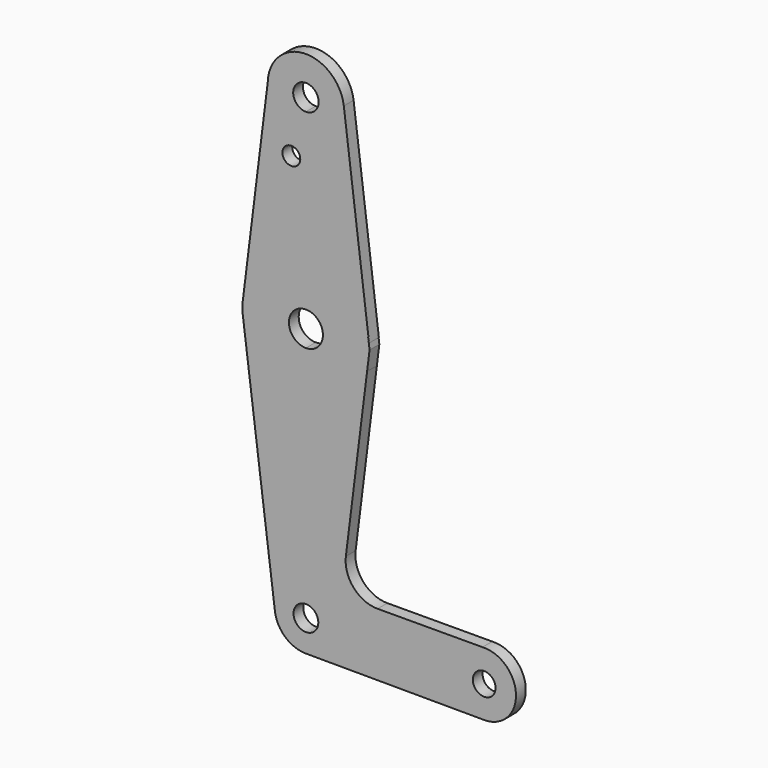
from build123d import *

# Parameters (mm, degrees)
F0_R     = 2.2225
F1_DEPTH = 3.048


# Not quite as in the source:
# - ends of sketch curves that miss each other by under 0.0002 mm in the source are joined


with BuildPart() as f1:
    # F0 (on Front) → F1 (new body)
    with BuildSketch(Plane.XZ):
        with BuildLine():
            Line((0, 104.775), (0, 79.375))
            ThreePointArc((0, 79.375), (9.9062001273, 75.9049515935), (15.4816923534, 67.0118124772))
            ThreePointArc((15.4816923534, 67.0118124772), (15.634754331, 66.2513782015), (15.7504882737, 65.484375))
            Line((15.7504882737, 65.484375), (9.4502929642, 115.490625))
            ThreePointArc((9.4502929642, 115.490625), (9.5063048942, 114.896483242), (9.525, 114.3))
            ThreePointArc((9.525, 114.3), (6.7351920908, 107.5648079092), (0, 104.775))
        make_face()
        with BuildLine():
            ThreePointArc((-15.3768101201, 67.4457997325), (-9.7307773134, 76.0430298523), (0, 79.375))
            Line((0, 79.375), (0, 104.775))
            ThreePointArc((0, 104.775), (-6.8164586923, 107.6470671207), (-9.5221925783, 114.5312433813))
            Line((-9.5221925783, 114.5312433813), (-15.3768101201, 67.4457997325))
        make_face()
        with Locations((-3.6322334781, 100.2735868096)):
            Circle(F0_R, mode=Mode.SUBTRACT)
        with BuildLine():
            ThreePointArc((-9.5221925783, 114.5312433813), (-6.8164586923, 107.6470671207), (0, 104.775))
            ThreePointArc((0, 104.775), (6.7351920908, 107.5648079092), (9.525, 114.3))
            ThreePointArc((9.525, 114.3), (9.5063048942, 114.896483242), (9.4502929642, 115.490625))
            ThreePointArc((9.4502929642, 115.490625), (-0.481036029, 123.8128454912), (-9.5221925783, 114.5312433813))
        make_face()
        with BuildLine():
            ThreePointArc((3.1731383542, 114.3), (2.2437476479, 112.0562523521), (0, 111.1268616458))
            ThreePointArc((0, 111.1268616458), (-2.2437476479, 116.5437476479), (3.1731383542, 114.3))
        make_face(mode=Mode.SUBTRACT)
        with BuildLine():
            Line((0, 59.2630050683), (0, 47.625))
            ThreePointArc((0, 47.625), (9.5420870367, 50.8128332563), (15.2519117252, 59.0960456714))
            Line((15.2519117252, 59.0960456714), (15.8668198703, 64.0095607934))
            Line((15.8668198703, 64.0095607934), (15.4816923534, 67.0118124772))
            ThreePointArc((15.4816923534, 67.0118124772), (9.9062001273, 75.9049515935), (0, 79.375))
            Line((0, 79.375), (0, 67.7369949317))
            ThreePointArc((0, 67.7369949317), (2.996007848, 66.496007848), (4.2369949317, 63.5))
            ThreePointArc((4.2369949317, 63.5), (2.996007848, 60.503992152), (0, 59.2630050683))
        make_face()
        with BuildLine():
            ThreePointArc((-15.7459735632, 61.4801134818), (-10.4868948341, 51.5819187057), (0, 47.625))
            Line((0, 47.625), (0, 59.2630050683))
            ThreePointArc((0, 59.2630050683), (-4.2369949317, 63.5), (0, 67.7369949317))
            Line((0, 67.7369949317), (0, 79.375))
            ThreePointArc((0, 79.375), (-9.7307773134, 76.0430298523), (-15.3768101201, 67.4457997325))
            Line((-15.3768101201, 67.4457997325), (-15.8748867846, 63.4400452066))
            ThreePointArc((-15.8748867846, 63.4400452066), (-15.8407712999, 62.4580836766), (-15.7459735632, 61.4801134818))
        make_face()
        with BuildLine():
            ThreePointArc((-7.7320952095, -0.9918697506), (-5.8524002287, 5.1496129461), (0, 7.7954539272))
            Line((0, 7.7954539272), (0, 47.625))
            ThreePointArc((0, 47.625), (-10.4868948341, 51.5819187057), (-15.7459735632, 61.4801134818))
            Line((-15.7459735632, 61.4801134818), (-7.7320952095, -0.9918697506))
        make_face()
        with BuildLine():
            Line((0, 47.625), (0, 7.7954539272))
            ThreePointArc((0, 7.7954539272), (5.5122183343, 5.5122183343), (7.7954539272, 0))
            Line((7.7954539272, 0), (36.5125, 0))
            ThreePointArc((36.5125, 0), (38.6941635505, 5.4657344444), (44.0398708389, 7.9268972695))
            Line((44.0398708389, 7.9268972695), (17.869380753, 7.8488082918))
            ThreePointArc((17.869380753, 7.8488082918), (11.8930439791, 10.5290526777), (9.9569931381, 16.7862100471))
            Line((9.9569931381, 16.7862100471), (15.2519117252, 59.0960456714))
            ThreePointArc((15.2519117252, 59.0960456714), (9.5420870367, 50.8128332563), (0, 47.625))
        make_face()
        with BuildLine():
            Line((36.5125, 0), (7.7954539272, 0))
            ThreePointArc((7.7954539272, 0), (5.5122183343, -5.5122183343), (0, -7.7954539272))
            Line((0, -7.7954539272), (43.9269950713, -7.9202507596))
            ThreePointArc((43.9269950713, -7.9202507596), (38.6553793104, -5.4245992768), (36.5125, 0))
        make_face()
        with BuildLine():
            ThreePointArc((3.0872431229, 0), (-2.1830105474, -2.1830105474), (0, 3.0872431229))
            Line((0, 3.0872431229), (0, 7.7954539272))
            ThreePointArc((0, 7.7954539272), (-5.8524002287, 5.1496129461), (-7.7320952095, -0.9918697506))
            ThreePointArc((-7.7320952095, -0.9918697506), (-5.1496129461, -5.8524002287), (0, -7.7954539272))
            ThreePointArc((0, -7.7954539272), (5.5122183343, -5.5122183343), (7.7954539272, 0))
            Line((7.7954539272, 0), (3.0872431229, 0))
        make_face()
        with BuildLine():
            Line((0, 7.7954539272), (0, 3.0872431229))
            ThreePointArc((0, 3.0872431229), (2.1830105474, 2.1830105474), (3.0872431229, 0))
            Line((3.0872431229, 0), (7.7954539272, 0))
            ThreePointArc((7.7954539272, 0), (5.5122183343, 5.5122183343), (0, 7.7954539272))
        make_face()
        with BuildLine():
            ThreePointArc((44.0398708389, 7.9268972695), (38.6941635505, 5.4657344444), (36.5125, 0))
            ThreePointArc((36.5125, 0), (38.6553793104, -5.4245992768), (43.9269950713, -7.9202507596))
            Line((43.9269950713, -7.9202507596), (44.9280052412, -7.9230939184))
            ThreePointArc((44.9280052412, -7.9230939184), (50.2291899455, -5.4410357308), (52.3875, 0))
            ThreePointArc((52.3875, 0), (49.9157344444, 5.7558364495), (44.0398708389, 7.9268972695))
        make_face()
        with BuildLine():
            ThreePointArc((47.2789731749, 0), (44.45, -2.8289731749), (41.6210268251, 0))
            ThreePointArc((41.6210268251, 0), (44.45, 2.8289731749), (47.2789731749, 0))
        make_face(mode=Mode.SUBTRACT)
    extrude(amount=F1_DEPTH)


solid = f1.part
